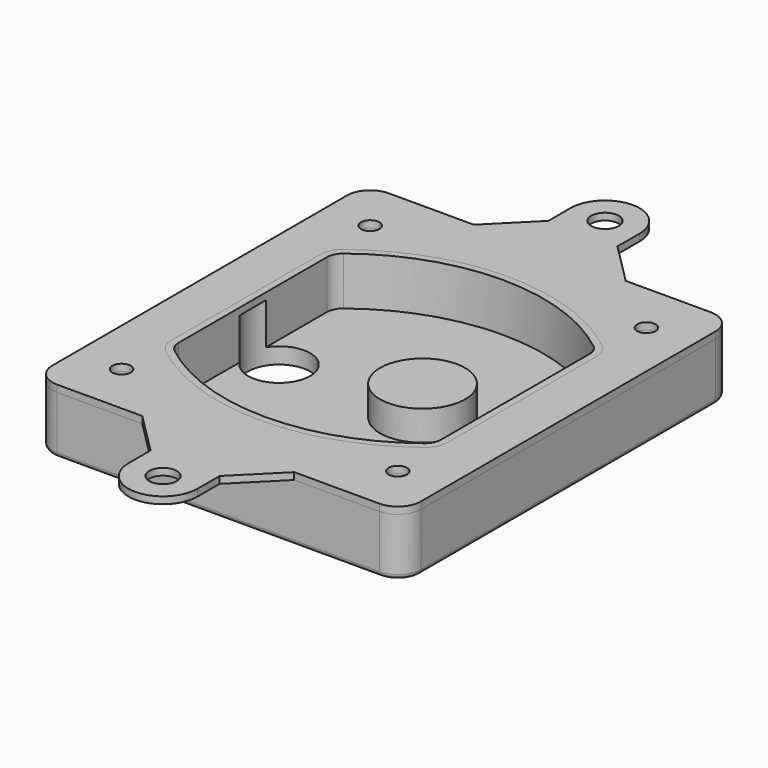
from build123d import *

# Parameters (mm, degrees)
F0_R      = 4
F1_DEPTH  = 25
F2_DEPTH  = 3
F3_DEPTH  = 18
F5_DEPTH  = 2
F7_DEPTH  = 20
F8_DEPTH  = 16
F9_DEPTH  = 25
F6_R      = 6
F6_R_2    = 4
F10_DEPTH = 6
F12_DEPTH = 9
F14_R     = 2
F15_R     = 6
F15_R_2   = 4
F16_DEPTH = 3


# Not quite as in the source:
# - a feature of the source that left no trace in its solid (it failed there, or was rolled back) is left out


with BuildPart() as f1:
    # F0 (on Top) → F1 (new body)
    with BuildSketch(Plane.XY):
        with BuildLine():
            ThreePointArc((-80, -80), (-77.0710678119, -87.0710678119), (-70, -90))
            Line((-70, -90), (70, -90))
            ThreePointArc((70, -90), (77.0710678119, -87.0710678119), (80, -80))
            Line((80, -80), (80, 80))
            ThreePointArc((80, 80), (77.0710678119, 87.0710678119), (70, 90))
            Line((70, 90), (-70, 90))
            ThreePointArc((-70, 90), (-77.0710678119, 87.0710678119), (-80, 80))
            Line((-80, 80), (-80, -80))
        make_face()
        with Locations((-60, -67.5)):
            Circle(F0_R, mode=Mode.SUBTRACT)
        with Locations((60, -67.5)):
            Circle(F0_R, mode=Mode.SUBTRACT)
        with Locations((-60, 67.5)):
            Circle(F0_R, mode=Mode.SUBTRACT)
        with BuildLine():
            ThreePointArc((-64, 40.2934422872), (-62.5820384798, 46.4328484224), (-58.6153846154, 51.3286200352))
            ThreePointArc((-58.6153846154, 51.3286200352), (0, 71.5), (58.6153846154, 51.3286200352))
            ThreePointArc((58.6153846154, 51.3286200352), (62.5820384798, 46.4328484224), (64, 40.2934422872))
            Line((64, 40.2934422872), (64, -40.2934422872))
            ThreePointArc((64, -40.2934422872), (62.5820384798, -46.4328484224), (58.6153846154, -51.3286200352))
            ThreePointArc((58.6153846154, -51.3286200352), (0, -71.5), (-58.6153846154, -51.3286200352))
            ThreePointArc((-58.6153846154, -51.3286200352), (-62.5820384798, -46.4328484224), (-64, -40.2934422872))
            Line((-64, -40.2934422872), (-64, 40.2934422872))
        make_face(mode=Mode.SUBTRACT)
        with Locations((60, 67.5)):
            Circle(F0_R, mode=Mode.SUBTRACT)
        with BuildLine():
            ThreePointArc((58.6153846154, 51.3286200352), (0, 71.5), (-58.6153846154, 51.3286200352))
            ThreePointArc((-58.6153846154, 51.3286200352), (-62.5820384798, 46.4328484224), (-64, 40.2934422872))
            Line((-64, 40.2934422872), (-64, -40.2934422872))
            ThreePointArc((-64, -40.2934422872), (-62.5820384798, -46.4328484224), (-58.6153846154, -51.3286200352))
            ThreePointArc((-58.6153846154, -51.3286200352), (0, -71.5), (58.6153846154, -51.3286200352))
            ThreePointArc((58.6153846154, -51.3286200352), (62.5820384798, -46.4328484224), (64, -40.2934422872))
            Line((64, -40.2934422872), (64, 40.2934422872))
            ThreePointArc((64, 40.2934422872), (62.5820384798, 46.4328484224), (58.6153846154, 51.3286200352))
        make_face()
        with BuildLine():
            Line((-60, -40.2934422872), (-60, 40.2934422872))
            ThreePointArc((-60, 40.2934422872), (-58.9871703427, 44.6787323838), (-56.1538461538, 48.1757121072))
            ThreePointArc((-56.1538461538, 48.1757121072), (0, 67.5), (56.1538461538, 48.1757121072))
            ThreePointArc((56.1538461538, 48.1757121072), (58.9871703427, 44.6787323838), (60, 40.2934422872))
            Line((60, 40.2934422872), (60, -40.2934422872))
            ThreePointArc((60, -40.2934422872), (58.9871703427, -44.6787323838), (56.1538461538, -48.1757121072))
            ThreePointArc((56.1538461538, -48.1757121072), (0, -67.5), (-56.1538461538, -48.1757121072))
            ThreePointArc((-56.1538461538, -48.1757121072), (-58.9871703427, -44.6787323838), (-60, -40.2934422872))
        make_face(mode=Mode.SUBTRACT)
        with BuildLine():
            ThreePointArc((-56.1538461538, 48.1757121072), (-58.9871703427, 44.6787323838), (-60, 40.2934422872))
            Line((-60, 40.2934422872), (-60, -40.2934422872))
            ThreePointArc((-60, -40.2934422872), (-58.9871703427, -44.6787323838), (-56.1538461538, -48.1757121072))
            ThreePointArc((-56.1538461538, -48.1757121072), (0, -67.5), (56.1538461538, -48.1757121072))
            ThreePointArc((56.1538461538, -48.1757121072), (58.9871703427, -44.6787323838), (60, -40.2934422872))
            Line((60, -40.2934422872), (60, 40.2934422872))
            ThreePointArc((60, 40.2934422872), (58.9871703427, 44.6787323838), (56.1538461538, 48.1757121072))
            ThreePointArc((56.1538461538, 48.1757121072), (0, 67.5), (-56.1538461538, 48.1757121072))
        make_face()
        with BuildLine():
            ThreePointArc((54.3076923077, 45.8110311612), (56.2910192399, 43.3631453548), (57, 40.2934422872))
            Line((57, 40.2934422872), (57, -40.2934422872))
            ThreePointArc((57, -40.2934422872), (56.2910192399, -43.3631453548), (54.3076923077, -45.8110311612))
            ThreePointArc((54.3076923077, -45.8110311612), (0, -64.5), (-54.3076923077, -45.8110311612))
            ThreePointArc((-54.3076923077, -45.8110311612), (-56.2910192399, -43.3631453548), (-57, -40.2934422872))
            Line((-57, -40.2934422872), (-57, 40.2934422872))
            ThreePointArc((-57, 40.2934422872), (-56.2910192399, 43.3631453548), (-54.3076923077, 45.8110311612))
            ThreePointArc((-54.3076923077, 45.8110311612), (0, 64.5), (54.3076923077, 45.8110311612))
        make_face(mode=Mode.SUBTRACT)
        with BuildLine():
            Line((57, -40.2934422872), (57, 40.2934422872))
            ThreePointArc((57, 40.2934422872), (56.2910192399, 43.3631453548), (54.3076923077, 45.8110311612))
            ThreePointArc((54.3076923077, 45.8110311612), (0, 64.5), (-54.3076923077, 45.8110311612))
            ThreePointArc((-54.3076923077, 45.8110311612), (-56.2910192399, 43.3631453548), (-57, 40.2934422872))
            Line((-57, 40.2934422872), (-57, -40.2934422872))
            ThreePointArc((-57, -40.2934422872), (-56.2910192399, -43.3631453548), (-54.3076923077, -45.8110311612))
            ThreePointArc((-54.3076923077, -45.8110311612), (0, -64.5), (54.3076923077, -45.8110311612))
            ThreePointArc((54.3076923077, -45.8110311612), (56.2910192399, -43.3631453548), (57, -40.2934422872))
        make_face()
    extrude(amount=-F1_DEPTH)

    # F0 (on Top) → F2 (join)
    with BuildSketch(Plane.XY):
        with BuildLine():
            ThreePointArc((-56.1538461538, 48.1757121072), (-58.9871703427, 44.6787323838), (-60, 40.2934422872))
            Line((-60, 40.2934422872), (-60, -40.2934422872))
            ThreePointArc((-60, -40.2934422872), (-58.9871703427, -44.6787323838), (-56.1538461538, -48.1757121072))
            ThreePointArc((-56.1538461538, -48.1757121072), (0, -67.5), (56.1538461538, -48.1757121072))
            ThreePointArc((56.1538461538, -48.1757121072), (58.9871703427, -44.6787323838), (60, -40.2934422872))
            Line((60, -40.2934422872), (60, 40.2934422872))
            ThreePointArc((60, 40.2934422872), (58.9871703427, 44.6787323838), (56.1538461538, 48.1757121072))
            ThreePointArc((56.1538461538, 48.1757121072), (0, 67.5), (-56.1538461538, 48.1757121072))
        make_face()
        with BuildLine():
            ThreePointArc((54.3076923077, 45.8110311612), (56.2910192399, 43.3631453548), (57, 40.2934422872))
            Line((57, 40.2934422872), (57, -40.2934422872))
            ThreePointArc((57, -40.2934422872), (56.2910192399, -43.3631453548), (54.3076923077, -45.8110311612))
            ThreePointArc((54.3076923077, -45.8110311612), (0, -64.5), (-54.3076923077, -45.8110311612))
            ThreePointArc((-54.3076923077, -45.8110311612), (-56.2910192399, -43.3631453548), (-57, -40.2934422872))
            Line((-57, -40.2934422872), (-57, 40.2934422872))
            ThreePointArc((-57, 40.2934422872), (-56.2910192399, 43.3631453548), (-54.3076923077, 45.8110311612))
            ThreePointArc((-54.3076923077, 45.8110311612), (0, 64.5), (54.3076923077, 45.8110311612))
        make_face(mode=Mode.SUBTRACT)
    extrude(amount=F2_DEPTH)

    # F0 (on Top) → F3 (cut)
    with BuildSketch(Plane.XY):
        with BuildLine():
            Line((57, -40.2934422872), (57, 40.2934422872))
            ThreePointArc((57, 40.2934422872), (56.2910192399, 43.3631453548), (54.3076923077, 45.8110311612))
            ThreePointArc((54.3076923077, 45.8110311612), (0, 64.5), (-54.3076923077, 45.8110311612))
            ThreePointArc((-54.3076923077, 45.8110311612), (-56.2910192399, 43.3631453548), (-57, 40.2934422872))
            Line((-57, 40.2934422872), (-57, -40.2934422872))
            ThreePointArc((-57, -40.2934422872), (-56.2910192399, -43.3631453548), (-54.3076923077, -45.8110311612))
            ThreePointArc((-54.3076923077, -45.8110311612), (0, -64.5), (54.3076923077, -45.8110311612))
            ThreePointArc((54.3076923077, -45.8110311612), (56.2910192399, -43.3631453548), (57, -40.2934422872))
        make_face()
    extrude(amount=-F3_DEPTH, mode=Mode.SUBTRACT)

    # F4 (on face) → F5 (cut)
    with BuildSketch(Plane.XY.offset(3)):
        with BuildLine():
            Line((23, -39.2465276821), (23, 39.2465276821))
            ThreePointArc((23, 39.2465276821), (21.7633659499, 42.89486221), (18.5632183908, 45.0393118368))
            ThreePointArc((18.5632183908, 45.0393118368), (0, 47.5), (-18.5632183908, 45.0393118368))
            ThreePointArc((-18.5632183908, 45.0393118368), (-21.7633659499, 42.89486221), (-23, 39.2465276821))
            Line((-23, 39.2465276821), (-23, -39.2465276821))
            ThreePointArc((-23, -39.2465276821), (-21.7633659499, -42.89486221), (-18.5632183908, -45.0393118368))
            ThreePointArc((-18.5632183908, -45.0393118368), (0, -47.5), (18.5632183908, -45.0393118368))
            ThreePointArc((18.5632183908, -45.0393118368), (21.7633659499, -42.89486221), (23, -39.2465276821))
        make_face()
        with BuildLine():
            ThreePointArc((18.0421455939, 43.1083837852), (20.1755772999, 41.6787507007), (21, 39.2465276821))
            Line((21, 39.2465276821), (21, -39.2465276821))
            ThreePointArc((21, -39.2465276821), (20.1755772999, -41.6787507007), (18.0421455939, -43.1083837852))
            ThreePointArc((18.0421455939, -43.1083837852), (0, -45.5), (-18.0421455939, -43.1083837852))
            ThreePointArc((-18.0421455939, -43.1083837852), (-20.1755772999, -41.6787507007), (-21, -39.2465276821))
            Line((-21, -39.2465276821), (-21, 39.2465276821))
            ThreePointArc((-21, 39.2465276821), (-20.1755772999, 41.6787507007), (-18.0421455939, 43.1083837852))
            ThreePointArc((-18.0421455939, 43.1083837852), (0, 45.5), (18.0421455939, 43.1083837852))
        make_face(mode=Mode.SUBTRACT)
    extrude(amount=-F5_DEPTH, mode=Mode.SUBTRACT)

    # F6 (on face) → F7 (join)
    with BuildSketch(Plane(origin=(0, 0, -25), x_dir=(1, 0, 0), z_dir=(0, 0, -1))):
        with BuildLine():
            ThreePointArc((3.28842436, 0), (16.7567035675, 13.4682792075), (30.224982775, 0))
            Line((30.224982775, 0), (35.224982775, 0))
            ThreePointArc((35.224982775, 0), (16.7567035675, 18.4682792075), (-1.71157564, 0))
            Line((-1.71157564, 0), (3.28842436, 0))
        make_face()
        with BuildLine():
            Line((3.28842436, 0), (30.224982775, 0))
            ThreePointArc((30.224982775, 0), (16.7567035675, 13.4682792075), (3.28842436, 0))
        make_face()
        with BuildLine():
            ThreePointArc((3.28842436, 0), (16.7567035675, -13.4682792075), (30.224982775, 0))
            Line((30.224982775, 0), (3.28842436, 0))
        make_face()
        with BuildLine():
            Line((35.224982775, 0), (30.224982775, 0))
            ThreePointArc((30.224982775, 0), (16.7567035675, -13.4682792075), (3.28842436, 0))
            Line((3.28842436, 0), (-1.71157564, 0))
            ThreePointArc((-1.71157564, 0), (16.7567035675, -18.4682792075), (35.224982775, 0))
        make_face()
    extrude(amount=-F7_DEPTH)

    # F6 (on face) → F8 (cut)
    with BuildSketch(Plane(origin=(0, 0, -25), x_dir=(1, 0, 0), z_dir=(0, 0, -1))):
        with BuildLine():
            Line((3.28842436, 0), (30.224982775, 0))
            ThreePointArc((30.224982775, 0), (16.7567035675, 13.4682792075), (3.28842436, 0))
        make_face()
        with BuildLine():
            ThreePointArc((3.28842436, 0), (16.7567035675, -13.4682792075), (30.224982775, 0))
            Line((30.224982775, 0), (3.28842436, 0))
        make_face()
    extrude(amount=-F8_DEPTH, mode=Mode.SUBTRACT)

    # F6 (on face) → F9 (cut)
    with BuildSketch(Plane(origin=(0, 0, -25), x_dir=(1, 0, 0), z_dir=(0, 0, -1))):
        with BuildLine():
            Line((-59.0318229325, 0), (-32.0952645175, 0))
            ThreePointArc((-32.0952645175, 0), (-45.563543725, 13.4682792075), (-59.0318229325, 0))
        make_face()
        with BuildLine():
            ThreePointArc((-59.0318229325, 0), (-45.563543725, -13.4682792075), (-32.0952645175, 0))
            Line((-32.0952645175, 0), (-59.0318229325, 0))
        make_face()
    extrude(amount=-F9_DEPTH, mode=Mode.SUBTRACT)

    # F6 (on face) → F10 (cut)
    with BuildSketch(Plane(origin=(0, 0, -25), x_dir=(1, 0, 0), z_dir=(0, 0, -1))):
        with Locations((60, -67.5)):
            Circle(F6_R)
        with Locations((60, -67.5)):
            Circle(F6_R_2, mode=Mode.SUBTRACT)
        with Locations((-60, -67.5)):
            Circle(F6_R)
        with Locations((-60, -67.5)):
            Circle(F6_R_2, mode=Mode.SUBTRACT)
        with Locations((-60, 67.5)):
            Circle(F6_R)
        with Locations((-60, 67.5)):
            Circle(F6_R_2, mode=Mode.SUBTRACT)
        with Locations((60, 67.5)):
            Circle(F6_R)
        with Locations((60, 67.5)):
            Circle(F6_R_2, mode=Mode.SUBTRACT)
    extrude(amount=-F10_DEPTH, mode=Mode.SUBTRACT)

    # F11 (on face) → F12 (cut, through all)
    with BuildSketch(Plane(origin=(0, 0, -9), x_dir=(1, 0, 0), z_dir=(0, 0, -1))):
        with BuildLine():
            Line((27.3984372721, -14.1485442653), (27.3984372721, -15.0940664053))
            ThreePointArc((27.3984372721, -15.0940664053), (27.475903284, -15.0391520481), (27.5530859277, -14.9838401226))
            ThreePointArc((27.5530859277, -14.9838401226), (27.7267756743, -14.8571482748), (27.8989788804, -14.728443154))
            ThreePointArc((27.8989788804, -14.728443154), (28.6543715524, -14.1252551626), (29.3771680347, -13.4833680332))
            ThreePointArc((29.3771680347, -13.4833680332), (30.0894740452, -12.7794588413), (30.7625777768, -12.0379742698))
            ThreePointArc((30.7625777768, -12.0379742698), (30.6440414845, -11.5954782507), (30.5678860614, -11.1437549604))
            ThreePointArc((30.5678860614, -11.1437549604), (30.4831955013, -11.1473467), (30.3984372721, -11.1485442653))
            ThreePointArc((30.3984372721, -11.1485442653), (28.2771169286, -12.0272239217), (27.3984372721, -14.1485442653))
        make_face()
        with BuildLine():
            ThreePointArc((37.6905631259, -6.728443154), (39.1958060597, -10.7902926705), (37.3915476096, -14.728443154))
            Line((37.3915476096, -14.728443154), (37.6905631259, -14.728443154))
            ThreePointArc((37.6905631259, -14.728443154), (39.8118834694, -13.8497634975), (40.6905631259, -11.728443154))
            Line((40.6905631259, -11.728443154), (40.6905631259, -9.728443154))
            ThreePointArc((40.6905631259, -9.728443154), (39.8118834694, -7.6071228104), (37.6905631259, -6.728443154))
        make_face()
        with BuildLine():
            ThreePointArc((30.7625777768, -12.0379742698), (31.2439734276, -11.4540974715), (31.7010455878, -10.8509897459))
            ThreePointArc((31.7010455878, -10.8509897459), (31.1488810727, -11.05316715), (30.5678860614, -11.1437549604))
            ThreePointArc((30.5678860614, -11.1437549604), (30.6440414845, -11.5954782507), (30.7625777768, -12.0379742698))
        make_face()
        with BuildLine():
            ThreePointArc((32.9048821405, -14.728443154), (33.1479898385, -14.8632336648), (33.3984372721, -14.9838401226))
            Line((33.3984372721, -14.9838401226), (37.097122848, -14.9838401226))
            ThreePointArc((37.097122848, -14.9838401226), (37.2465319962, -14.8586740986), (37.3915476096, -14.728443154))
            Line((37.3915476096, -14.728443154), (32.9048821405, -14.728443154))
        make_face()
        with BuildLine():
            Line((37.097122848, -14.9838401226), (33.3984372721, -14.9838401226))
            ThreePointArc((33.3984372721, -14.9838401226), (35.1063741518, -15.3971839704), (36.8492913953, -15.1732621))
            ThreePointArc((36.8492913953, -15.1732621), (36.9745109281, -15.0802569548), (37.097122848, -14.9838401226))
        make_face()
        with BuildLine():
            ThreePointArc((37.097122848, -14.9838401226), (36.9745109281, -15.0802569548), (36.8492913953, -15.1732621))
            ThreePointArc((36.8492913953, -15.1732621), (37.0995782353, -15.0853439985), (37.3446701732, -14.9838401226))
            Line((37.3446701732, -14.9838401226), (37.097122848, -14.9838401226))
        make_face()
    extrude(amount=F12_DEPTH, mode=Mode.SUBTRACT)

    # F14
    f14_edges = [f1.edges().sort_by_distance(p)[0] for p in [
        (0, -90, -25),
        (-77.071068, -87.071068, -25),
        (-80, 0, -25),
        (-77.071068, 87.071068, -25),
        (77.071068, -87.071068, -25),
        (0, 90, -25),
        (80, 0, -25),
        (77.071068, 87.071068, -25),
    ]]
    fillet(f14_edges, radius=F14_R)


with BuildPart() as f16:
    # F15 (on face) → F16 (new body, through all)
    with BuildSketch(Plane.XY):
        with BuildLine():
            Line((-15, 108), (-33, 90))
            Line((-33, 90), (33, 90))
            Line((33, 90), (15, 108))
            Line((15, 108), (15, 120))
            ThreePointArc((15, 120), (0, 135), (-15, 120))
            Line((-15, 120), (-15, 108))
        make_face()
        with Locations((0, 120)):
            Circle(F15_R, mode=Mode.SUBTRACT)
        with BuildLine():
            Line((33, -90), (-33, -90))
            Line((-33, -90), (-15, -108))
            Line((-15, -108), (-15, -120))
            ThreePointArc((-15, -120), (0, -135), (15, -120))
            Line((15, -120), (15, -108))
            Line((15, -108), (33, -90))
        make_face()
        with Locations((0, -120)):
            Circle(F15_R, mode=Mode.SUBTRACT)
        with BuildLine():
            Line((-33, 90), (-70, 90))
            ThreePointArc((-70, 90), (-77.0710678119, 87.0710678119), (-80, 80))
            Line((-80, 80), (-80, -80))
            ThreePointArc((-80, -80), (-77.0710678119, -87.0710678119), (-70, -90))
            Line((-70, -90), (-33, -90))
            Line((-33, -90), (33, -90))
            Line((33, -90), (70, -90))
            ThreePointArc((70, -90), (77.0710678119, -87.0710678119), (80, -80))
            Line((80, -80), (80, 80))
            ThreePointArc((80, 80), (77.0710678119, 87.0710678119), (70, 90))
            Line((70, 90), (33, 90))
            Line((33, 90), (-33, 90))
        make_face()
        with Locations((-60, -67.5)):
            Circle(F15_R_2, mode=Mode.SUBTRACT)
        with Locations((60, -67.5)):
            Circle(F15_R_2, mode=Mode.SUBTRACT)
        with Locations((-60, 67.5)):
            Circle(F15_R_2, mode=Mode.SUBTRACT)
        with BuildLine():
            ThreePointArc((-56.1538461538, 48.1757121072), (0, 67.5), (56.1538461538, 48.1757121072))
            ThreePointArc((56.1538461538, 48.1757121072), (58.9871703427, 44.6787323838), (60, 40.2934422872))
            Line((60, 40.2934422872), (60, -40.2934422872))
            ThreePointArc((60, -40.2934422872), (58.9871703427, -44.6787323838), (56.1538461538, -48.1757121072))
            ThreePointArc((56.1538461538, -48.1757121072), (0, -67.5), (-56.1538461538, -48.1757121072))
            ThreePointArc((-56.1538461538, -48.1757121072), (-58.9871703427, -44.6787323838), (-60, -40.2934422872))
            Line((-60, -40.2934422872), (-60, 40.2934422872))
            ThreePointArc((-60, 40.2934422872), (-58.9871703427, 44.6787323838), (-56.1538461538, 48.1757121072))
        make_face(mode=Mode.SUBTRACT)
        with Locations((60, 67.5)):
            Circle(F15_R_2, mode=Mode.SUBTRACT)
    extrude(amount=F16_DEPTH)


solid = Compound([f1.part, f16.part])
